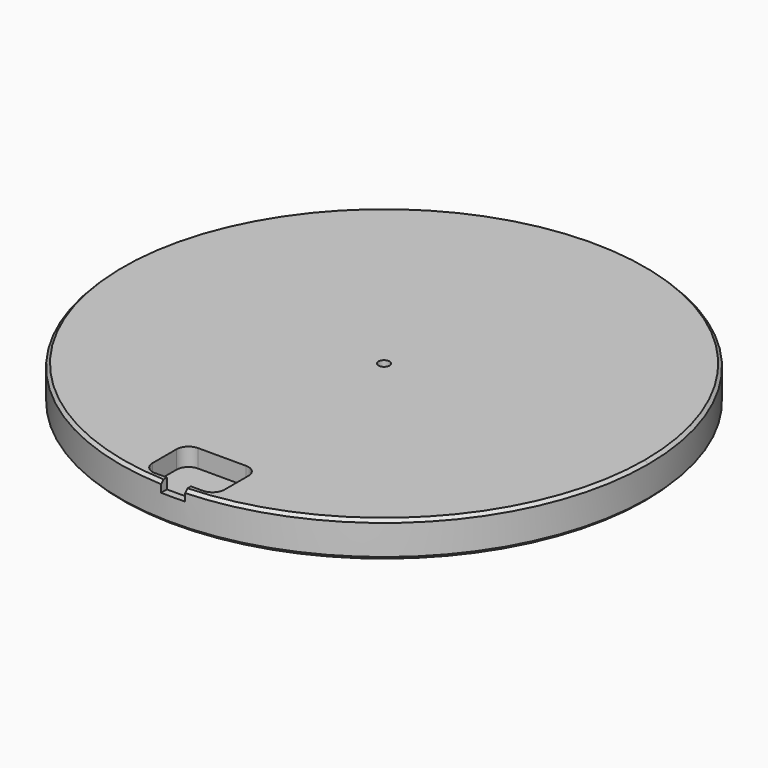
from build123d import *

# Parameters (mm, degrees)
F2_R     = 139.7
F2_R_2   = 2.9765625
F3_DEPTH = 19.05
F4_SIZE  = 1.5875
F6_DEPTH = 5.55625
F8_DEPTH = 9.525


# Not quite as in the source:
# - a variable given as a bare number and used for a length is read in inches; the dataset says mm whatever the document's units were


with BuildPart() as f3:
    # F2 (on Top) → F3 (new body)
    with BuildSketch(Plane.XY):
        Circle(F2_R)
        Circle(F2_R_2, mode=Mode.SUBTRACT)
    extrude(amount=F3_DEPTH)

    # F4
    f4_edges = [f3.edges().sort_by_distance(p)[0] for p in [
        (-139.7, 0, 19.05),
        (-139.7, 0, 0),
    ]]
    chamfer(f4_edges, length=F4_SIZE)

    # F5 (on face) → F6 (cut)
    with BuildSketch(Plane.XY.offset(19.05)):
        with BuildLine():
            Line((6.35, -137.9664457622), (6.35, -114.2999987969))
            ThreePointArc((6.35, -114.2999987969), (-6.016e-07, -107.95), (-6.35, -114.3))
            Line((-6.35, -114.3), (-6.35, -137.9664457622))
            ThreePointArc((-6.35, -137.9664457622), (0, -138.1125), (6.35, -137.9664457622))
        make_face()
        with BuildLine():
            Line((6.35, -143.818885088), (6.35, -137.9664457622))
            ThreePointArc((6.35, -137.9664457622), (0, -138.1125), (-6.35, -137.9664457622))
            Line((-6.35, -137.9664457622), (-6.35, -143.818885088))
            Line((-6.35, -143.818885088), (6.35, -143.818885088))
        make_face()
    extrude(amount=-F6_DEPTH, mode=Mode.SUBTRACT)

    # F7 (on face) → F8 (cut)
    with BuildSketch(Plane.XY.offset(19.05)):
        with BuildLine():
            Line((12.7, -107.15625), (-12.7, -107.15625))
            ThreePointArc((-12.7, -107.15625), (-17.1901280605, -109.0161219395), (-19.05, -113.50625))
            Line((-19.05, -113.50625), (-19.05, -129.38125))
            ThreePointArc((-19.05, -129.38125), (-17.1901280605, -133.8713780605), (-12.7, -135.73125))
            Line((-12.7, -135.73125), (-6.35, -135.73125))
            Line((-6.35, -135.73125), (-6.35, -114.3))
            ThreePointArc((-6.35, -114.3), (-6.016e-07, -107.95), (6.35, -114.2999987969))
            Line((6.35, -114.2999987969), (6.35, -135.73125))
            Line((6.35, -135.73125), (12.7, -135.73125))
            ThreePointArc((12.7, -135.73125), (17.1901280605, -133.8713780605), (19.05, -129.38125))
            Line((19.05, -129.38125), (19.05, -113.50625))
            ThreePointArc((19.05, -113.50625), (17.1901280605, -109.0161219395), (12.7, -107.15625))
        make_face()
        with BuildLine():
            Line((-6.35, -114.3), (-6.35, -135.73125))
            Line((-6.35, -135.73125), (6.35, -135.73125))
            Line((6.35, -135.73125), (6.35, -114.2999987969))
            ThreePointArc((6.35, -114.2999987969), (-6.016e-07, -107.95), (-6.35, -114.3))
        make_face()
    extrude(amount=-F8_DEPTH, mode=Mode.SUBTRACT)


solid = f3.part
